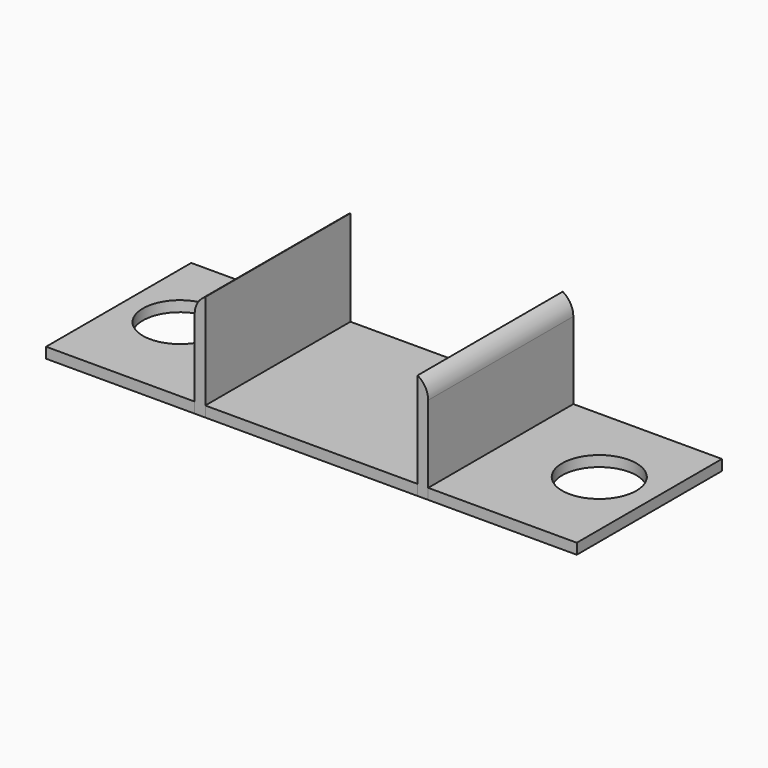
from build123d import *

# Parameters (mm, degrees)
F0_W          = 2.54
F0_H          = 43.4209238519
F1_DEPTH      = 25.4
F0_W_2        = 35.56
F0_R          = 8.89
F2_DEPTH      = 2.54
F0_W_3        = 50.8
F3_T1_DEPTH   = 65.417969108
F3_2_T1_DEPTH = 65.417969108


# Not quite as in the source:
# - a fillet or chamfer that OpenCascade refuses, or shapes differently, is made with other operations: its cross-section is extruded or revolved along the edge and cut away or added


with BuildPart() as f1:
    # F0 (on Top) → F1 (new body)
    with BuildSketch(Plane.XY):
        with Locations((4.3516923602, -49.3432171643)):
            Rectangle(F0_W, F0_H)
    extrude(amount=F1_DEPTH)

    # F3: fillet of radius 5.08 on 1 edges, made by hand

    # F3_s2 → F3_t1 (cut)
    with BuildSketch(Plane.XZ.offset(16.6342326103)):
        with BuildLine():
            ThreePointArc((3.0816923602, 21.0005909488), (3.762283309, 23.5405909488), (5.6216923602, 25.4))
            Line((5.6216923602, 25.4), (3.0816923602, 25.4))
            Line((3.0816923602, 25.4), (3.0816923602, 21.0005909488))
        make_face()
    extrude(amount=F3_T1_DEPTH, mode=Mode.SUBTRACT)


with BuildPart() as f1b:
    # F0 (on Top) → F1, piece 2 (new body)
    with BuildSketch(Plane.XY):
        with Locations((57.6916923602, -49.3432171643)):
            Rectangle(F0_W, F0_H)
    extrude(amount=F1_DEPTH)

    # F3#2: fillet of radius 5.08 on 1 edges, made by hand

    # F3_2_s2 → F3_2_t1 (cut)
    with BuildSketch(Plane.XZ.offset(16.6342326103)):
        with BuildLine():
            ThreePointArc((58.9616923602, 21.0005909488), (58.2811014114, 23.5405909488), (56.4216923602, 25.4))
            Line((56.4216923602, 25.4), (58.9616923602, 25.4))
            Line((58.9616923602, 25.4), (58.9616923602, 21.0005909488))
        make_face()
    extrude(amount=F3_2_T1_DEPTH, mode=Mode.SUBTRACT)


with BuildPart() as f2:
    # F0 (on Top) → F2 (new body)
    with BuildSketch(Plane.XY):
        with Locations((-14.6983076398, -49.3432171643)):
            Rectangle(F0_W_2, F0_H)
        with Locations((-19.1433076398, -47.6529405909)):
            Circle(F0_R, mode=Mode.SUBTRACT)
    extrude(amount=F2_DEPTH)


with BuildPart() as f2b:
    # F0 (on Top) → F2, piece 2 (new body)
    with BuildSketch(Plane.XY):
        with Locations((31.0216923602, -49.3432171643)):
            Rectangle(F0_W_3, F0_H)
    extrude(amount=F2_DEPTH)


with BuildPart() as f2c:
    # F0 (on Top) → F2, piece 3 (new body)
    with BuildSketch(Plane.XY):
        with Locations((76.7416923602, -49.3432171643)):
            Rectangle(F0_W_2, F0_H)
        with Locations((81.1866923602, -47.6529405909)):
            Circle(F0_R, mode=Mode.SUBTRACT)
    extrude(amount=F2_DEPTH)


solid = Compound([f1.part, f1b.part, f2.part, f2b.part, f2c.part])
